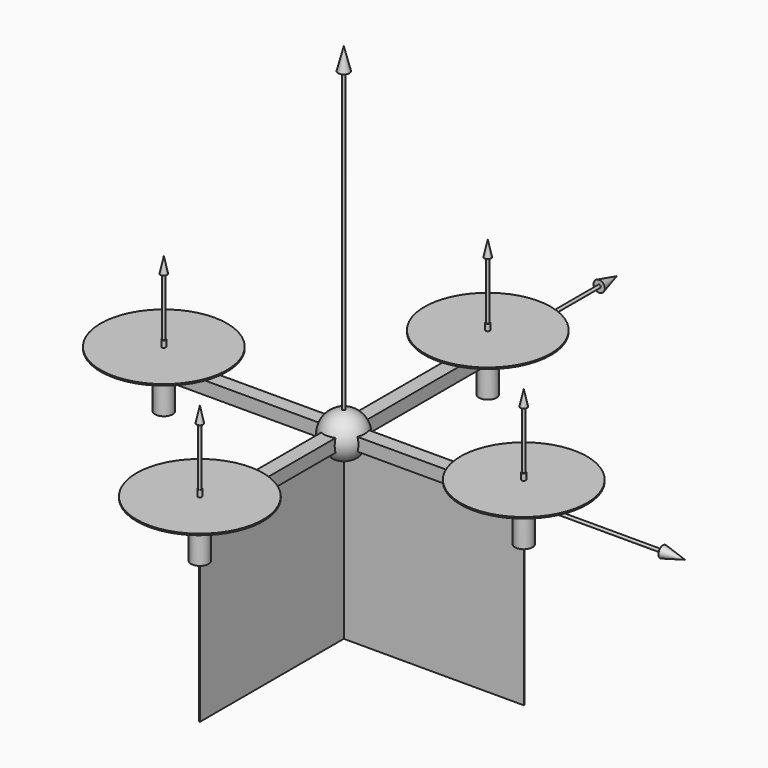
from build123d import *

# Parameters (mm, degrees)
F1_DEPTH  = 9
F4_R      = 12.1675169792
F5_DEPTH  = 62.5
F9_COUNT  = 2
F9_ANGLE  = 90
F10_COUNT = 2
F10_ANGLE = 270
F11_R     = 2.7870982488
F12_DEPTH = 25
F14_R     = 87.5
F15_DEPTH = 2
F16_D     = 5
F17_COUNT = 4
F18_R     = 2.0523071478
F19_DEPTH = 80
F23_COUNT = 4
F25_DEPTH = 250


with BuildPart() as f1:
    # F0 (on Top) → F1 (new body, symmetric)
    with BuildSketch(Plane.XY):
        Polygon((0, -9.9708658014), (0, 0), (-9.9708658014, 0), (-9.9708658014, -10), (0.0291341986, -10), (0.0291341986, -9.9708658014), align=None)
        Polygon((-9.9708658014, -10), (-9.9708658014, 0), (-10, 0), (-10, 10), (-249.9708658014, 10), (-249.9708658014, 7.6838978223), (-249.9708658014, -7.6838978223), (-249.9708658014, -10), align=None)
        Polygon((-10, 0), (-9.9708658014, 0), (-9.9708658014, 0.0291341986), (0, 0.0291341986), (0, 10), (-10, 10), align=None)
        Polygon((10, 0), (0.0291341986, 0), (0.0291341986, -9.9708658014), (10.0291341986, -9.9708658014), (10.0291341986, 0.0291341986), (10, 0.0291341986), align=None)
        Polygon((0.0291341986, -10), (-9.9708658014, -10), (-9.9708658014, -249.9708658014), (-7.6547636237, -249.9708658014), (7.7130320208, -249.9708658014), (10.0291341986, -249.9708658014), (10.0291341986, -9.9708658014), (0.0291341986, -9.9708658014), align=None)
        Polygon((0.0291341986, 10), (0.0291341986, 0.0291341986), (10, 0.0291341986), (10, 10.0291341986), (0, 10.0291341986), (0, 10), align=None)
        with BuildLine():
            Line((-10, 10), (0, 10))
            Line((0, 10), (0, 10.0291341986))
            Line((0, 10.0291341986), (10, 10.0291341986))
            Line((10, 10.0291341986), (10, 249.2361068314))
            ThreePointArc((10, 249.2361068314), (0, 239.9708658014), (-10, 249.2361068314))
            Line((-10, 249.2361068314), (-10, 10))
        make_face()
        Polygon((10, 10.0291341986), (10, 0.0291341986), (10.0291341986, 0.0291341986), (10.0291341986, -9.9708658014), (250, -9.9708658014), (250, -7.6547636237), (250, 7.7130320208), (250, 10.0291341986), align=None)
        with BuildLine():
            ThreePointArc((10.0291341986, 250), (-0.3822242714, 260.0218480022), (-10, 249.2361068314))
            Line((-10, 249.2361068314), (-10, 250))
            Line((-10, 250), (-7.6838978223, 250))
            Line((-7.6838978223, 250), (7.6838978223, 250))
            Line((7.6838978223, 250), (10, 250))
            Line((10, 250), (10, 249.2361068314))
            ThreePointArc((10, 249.2361068314), (10.0218480022, 249.6177757286), (10.0291341986, 250))
        make_face()
        with BuildLine():
            Line((-10, 250), (-10, 249.2361068314))
            ThreePointArc((-10, 249.2361068314), (0, 239.9708658014), (10, 249.2361068314))
            Line((10, 249.2361068314), (10, 250))
            Line((10, 250), (7.6838978223, 250))
            Line((7.6838978223, 250), (-7.6838978223, 250))
            Line((-7.6838978223, 250), (-10, 250))
        make_face()
    extrude(amount=F1_DEPTH, both=True)

    # F2 (on Top) → F3 (revolve)
    with BuildSketch(Plane.XY):
        with BuildLine():
            Line((0, 0), (30, 0))
            ThreePointArc((30, 0), (0, 30), (-30, 0))
            Line((-30, 0), (0, 0))
        make_face()
    revolve(axis=Axis((154.5636355877, 0, 0), (1, 0, 0)))

    # F4 (on face) → F5 (join)
    with BuildSketch(Plane.XY.offset(9)):
        with Locations((0, 249.1697371006)):
            Circle(F4_R)
        with Locations((-249.1697371006, 0)):
            Circle(F4_R)
        with Locations((0, -249.1697371006)):
            Circle(F4_R)
        with Locations((249.1697371006, 0)):
            Circle(F4_R)
    extrude(amount=-F5_DEPTH)

    # F11 (on face) → F12 (join)
    with BuildSketch(Plane.XY.offset(9)):
        with Locations((0, 249.1697371006)):
            Circle(F11_R)
        with Locations((-249.1697371006, 0)):
            Circle(F11_R)
        with Locations((0, -249.1697371006)):
            Circle(F11_R)
        with Locations((249.1697371006, 0)):
            Circle(F11_R)
    extrude(amount=F12_DEPTH)


with BuildPart() as f8:
    # F7 (on Top) → F8 (revolve)
    with BuildSketch(Plane.XY):
        Polygon((-7.8473286703, 441.9736564159), (-2, 441.9736564159), (-2, 0), (0, 0), (0, 2), (0, 441.9736564159), (0, 472.5137352943), align=None)
    revolve(axis=Axis((0, 220.986828208, 0), (0, -1, 0)))


with BuildPart() as f9_1:
    # F9: instance of F8
    add(f8.part.rotate(Axis((15, 0, 0), (1, 0, 0)), 1 * F9_ANGLE / (F9_COUNT - 1)))


with BuildPart() as f8_1:
    add(f8.part)

    add(f9_1.part)  # F10 merges F9_1
    # F10: F9_1 ×2 about axis
    f10_axis = Axis((0, 160.3847742081, 0), (0, -1, 0))
    for i in range(1, F10_COUNT):
        add(f9_1.part.rotate(f10_axis, i * F10_ANGLE / (F10_COUNT - 1)))


with BuildPart() as f15:
    # F14 (on offset) → F15 (new body)
    with BuildSketch(Plane.XY.offset(25)):
        with Locations((0, 249.1697371006)):
            Circle(F14_R)
    extrude(amount=-F15_DEPTH)

    # F16 (through all)
    with Locations(Plane(origin=(0, 0, 9), x_dir=(1, 0, 0), z_dir=(0, 0, -1))):
        with Locations((0, -249.1697371006)):
            Hole(F16_D / 2)


with BuildPart() as f17_1:
    # F17: instance of F15
    add(f15.part.rotate(Axis((0, 0, 441.9736564159), (0, 0, -1)), 1 * 360 / F17_COUNT))


with BuildPart() as f17_2:
    # F17: instance of F15
    add(f15.part.rotate(Axis((0, 0, 441.9736564159), (0, 0, -1)), 2 * 360 / F17_COUNT))


with BuildPart() as f17_3:
    # F17: instance of F15
    add(f15.part.rotate(Axis((0, 0, 441.9736564159), (0, 0, -1)), 3 * 360 / F17_COUNT))


with BuildPart() as f19:
    # F18 (on face) → F19 (new body)
    with BuildSketch(Plane.XY.offset(34)):
        with Locations((0, 249.1697371006)):
            Circle(F18_R)
    extrude(amount=F19_DEPTH)

    # F21 (on line) → F22 (revolve)
    with BuildSketch(Plane.XZ.offset(-249.1697371006)):
        Polygon((4.6796025708, 114), (0, 135.8055919409), (0, 114), align=None)
    revolve(axis=Axis((0, 249.1697371006, 124.9027959704), (0, 0, 1)))


with BuildPart() as f23_1:
    # F23: instance of F19
    add(f19.part.rotate(Axis((0, 0, 441.9736564159), (0, 0, -1)), 1 * 360 / F23_COUNT))


with BuildPart() as f23_2:
    # F23: instance of F19
    add(f19.part.rotate(Axis((0, 0, 441.9736564159), (0, 0, -1)), 2 * 360 / F23_COUNT))


with BuildPart() as f23_3:
    # F23: instance of F19
    add(f19.part.rotate(Axis((0, 0, 441.9736564159), (0, 0, -1)), 3 * 360 / F23_COUNT))


with BuildPart() as f25:
    # F24 (on Top) → F25 (new body)
    with BuildSketch(Plane.XY):
        Polygon((0, -249.1697371006), (0, 0), (249.1697371006, 0), (249.1697371006, 1), (-1, 1), (-1, -249.1697371006), align=None)
    extrude(amount=-F25_DEPTH)


solid = Compound([f1.part, f8_1.part, f15.part, f17_1.part, f17_2.part, f17_3.part, f19.part, f23_1.part, f23_2.part, f23_3.part, f25.part])
